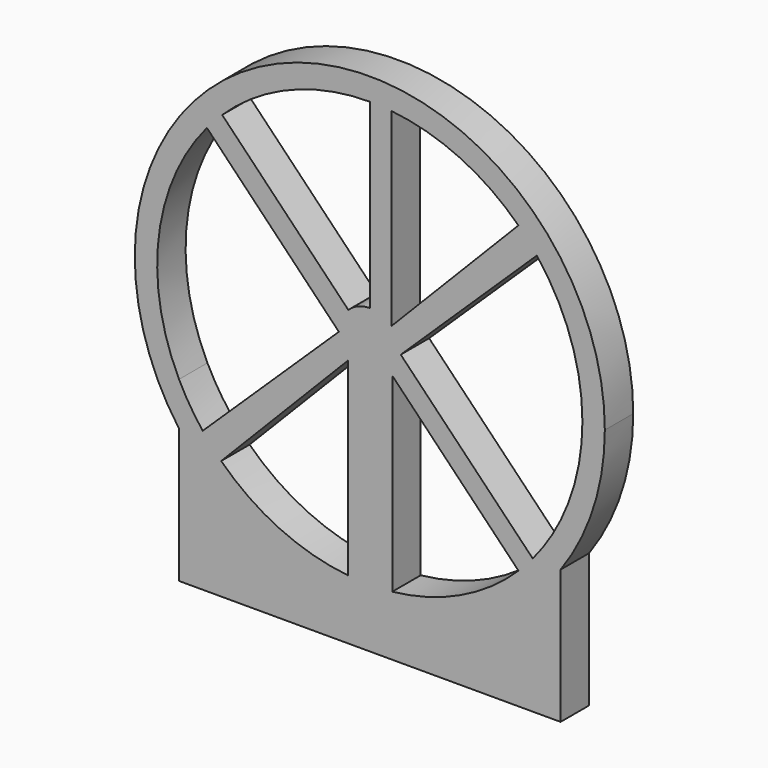
from build123d import *

# Parameters (mm, degrees)
F1_DEPTH = 7.62


# Not quite as in the source:
# - a feature names something its author has since deleted; it is built from what else it names


with BuildPart() as f1:
    # F0 (on Front) → F1 (new body)
    with BuildSketch(Plane.XZ):
        with BuildLine():
            ThreePointArc((10.3407477596, 18.5977799931), (17.6059784875, 5.3059692522), (20.1200594207, -9.6317416622))
            ThreePointArc((20.1200594207, -9.6317416622), (18.9331000604, -19.9720923089), (15.4339684141, -29.7745308699))
            Line((15.4339684141, -29.7745308699), (15.4339684141, -39.0992002321))
            ThreePointArc((15.4339684141, -39.0992002321), (22.5007653243, -25.1123260967), (24.9346453986, -9.6317416622))
            ThreePointArc((24.9346453986, -9.6317416622), (-40.9946586007, 38.3830978282), (-66.4621167465, -39.0992002321))
            Line((-66.4621167465, -39.0992002321), (-66.4621167465, -29.7745308699))
            ThreePointArc((-66.4621167465, -29.7745308699), (-70.8175510234, -4.1482087801), (-60.473849015, 19.6989298396))
            ThreePointArc((-60.473849015, 19.6989298396), (-58.8829140283, 21.49693763), (-57.1996202187, 23.2087869508))
            ThreePointArc((-57.1996202187, 23.2087869508), (-42.5995223376, 32.6832865075), (-25.5140741662, 36.0023919246))
            ThreePointArc((-25.5140741662, 36.0023919246), (-23.1888304756, 35.9431131373), (-20.869627773, 35.7654307819))
            ThreePointArc((-20.869627773, 35.7654307819), (-6.1592475305, 31.6945796612), (6.3859014459, 23.0005384324))
            ThreePointArc((6.3859014459, 23.0005384324), (8.4347729102, 20.8633387673), (10.3407477596, 18.5977799931))
        make_face()
        with BuildLine():
            Line((15.4339684141, -39.0992002321), (15.4339684141, -29.7745308699))
            ThreePointArc((15.4339684141, -29.7745308699), (12.7227075108, -34.5400269346), (9.459491795, -38.9459674269))
            ThreePointArc((9.459491795, -38.9459674269), (7.971092144, -40.635254131), (6.4011850797, -42.2490741021))
            ThreePointArc((6.4011850797, -42.2490741021), (-6.064908215, -50.9137485421), (-20.6835588609, -55.0094924892))
            ThreePointArc((-20.6835588609, -55.0094924892), (-25.4205342826, -55.265779381), (-30.1585205594, -55.0289141064))
            ThreePointArc((-30.1585205594, -55.0289141064), (-44.8689008019, -50.9580629857), (-57.4140497783, -42.2640217569))
            ThreePointArc((-57.4140497783, -42.2640217569), (-59.4700632753, -40.1188693041), (-61.3821167465, -37.8444634324))
            ThreePointArc((-61.3821167465, -37.8444634324), (-64.1334823406, -33.9425512021), (-66.4621167465, -29.7745308699))
            Line((-66.4621167465, -29.7745308699), (-66.4621167465, -39.0992002321))
            ThreePointArc((-66.4621167465, -39.0992002321), (-25.5140741662, -60.0804612271), (15.4339684141, -39.0992002321))
        make_face()
        with BuildLine():
            Line((15.4339684141, -55.2114608665), (15.4339684141, -39.0992002321))
            ThreePointArc((15.4339684141, -39.0992002321), (-25.5140741662, -60.0804612271), (-66.4621167465, -39.0992002321))
            Line((-66.4621167465, -39.0992002321), (-66.4621167465, -58.9845308699))
            Line((-66.4621167465, -58.9845308699), (-66.4621167465, -67.8745308699))
            Line((-66.4621167465, -67.8745308699), (15.4339684141, -67.8745308699))
            Line((15.4339684141, -67.8745308699), (15.4339684141, -58.9845308699))
            Line((15.4339684141, -58.9845308699), (15.4339684141, -55.2114608665))
        make_face()
        with BuildLine():
            Line((-30.119077868, -4.8424361606), (-57.1996202187, 23.2087869508))
            ThreePointArc((-57.1996202187, 23.2087869508), (-58.8829140283, 21.49693763), (-60.473849015, 19.6989298396))
            Line((-60.473849015, 19.6989298396), (-32.1581321342, -9.6317416622))
            ThreePointArc((-32.1581321342, -9.6317416622), (-31.6271510436, -7.0290896739), (-30.119077868, -4.8424361606))
        make_face()
        with BuildLine():
            Line((-57.4140497783, -42.2640217569), (-30.1585205594, -14.3828072251))
            ThreePointArc((-30.1585205594, -14.3828072251), (-31.6378588353, -12.2090983718), (-32.1581321342, -9.6317416622))
            Line((-32.1581321342, -9.6317416622), (-61.3821167465, -37.8444634324))
            ThreePointArc((-61.3821167465, -37.8444634324), (-59.4700632753, -40.1188693041), (-57.4140497783, -42.2640217569))
        make_face()
        with BuildLine():
            Line((-20.6835588609, -55.0094924892), (-20.6835588609, -14.1934987981))
            ThreePointArc((-20.6835588609, -14.1934987981), (-25.3813532931, -16.2744738901), (-30.1585205594, -14.3828072251))
            Line((-30.1585205594, -14.3828072251), (-30.1585205594, -55.0289141064))
            ThreePointArc((-30.1585205594, -55.0289141064), (-25.4205342826, -55.265779381), (-20.6835588609, -55.0094924892))
        make_face()
        with BuildLine():
            Line((-18.8700161982, -9.6317416622), (10.3407477596, 18.5977799931))
            ThreePointArc((10.3407477596, 18.5977799931), (8.4347729102, 20.8633387673), (6.3859014459, 23.0005384324))
            Line((6.3859014459, 23.0005384324), (-20.869627773, -4.8806760994))
            ThreePointArc((-20.869627773, -4.8806760994), (-19.3902894971, -7.0543849527), (-18.8700161982, -9.6317416622))
        make_face()
        with BuildLine():
            Line((-20.869627773, -4.8806760994), (-20.869627773, 35.7654307819))
            ThreePointArc((-20.869627773, 35.7654307819), (-23.1888304756, 35.9431131373), (-25.5140741662, 36.0023919246))
            Line((-25.5140741662, 36.0023919246), (-25.5140741662, -2.9876836943))
            ThreePointArc((-25.5140741662, -2.9876836943), (-23.006370907, -3.4791055894), (-20.869627773, -4.8806760994))
        make_face()
        with BuildLine():
            ThreePointArc((-20.6835588609, -14.1934987981), (-19.340026467, -12.0862561334), (-18.8700161982, -9.6317416622))
            ThreePointArc((-18.8700161982, -9.6317416622), (-19.3902894971, -7.0543849527), (-20.869627773, -4.8806760994))
            ThreePointArc((-20.869627773, -4.8806760994), (-23.006370907, -3.4791055894), (-25.5140741662, -2.9876836943))
            ThreePointArc((-25.5140741662, -2.9876836943), (-27.9963194101, -3.4687906783), (-30.119077868, -4.8424361606))
            ThreePointArc((-30.119077868, -4.8424361606), (-31.6271510436, -7.0290896739), (-32.1581321342, -9.6317416622))
            ThreePointArc((-32.1581321342, -9.6317416622), (-31.6378588353, -12.2090983718), (-30.1585205594, -14.3828072251))
            ThreePointArc((-30.1585205594, -14.3828072251), (-25.3813532931, -16.2744738901), (-20.6835588609, -14.1934987981))
        make_face()
        with BuildLine():
            Line((9.459491795, -38.9459674269), (-18.8700161982, -9.6317416622))
            ThreePointArc((-18.8700161982, -9.6317416622), (-19.340026467, -12.0862561334), (-20.6835588609, -14.1934987981))
            Line((-20.6835588609, -14.1934987981), (6.4011850797, -42.2490741021))
            ThreePointArc((6.4011850797, -42.2490741021), (7.971092144, -40.635254131), (9.459491795, -38.9459674269))
        make_face()
    extrude(amount=F1_DEPTH)


solid = f1.part
